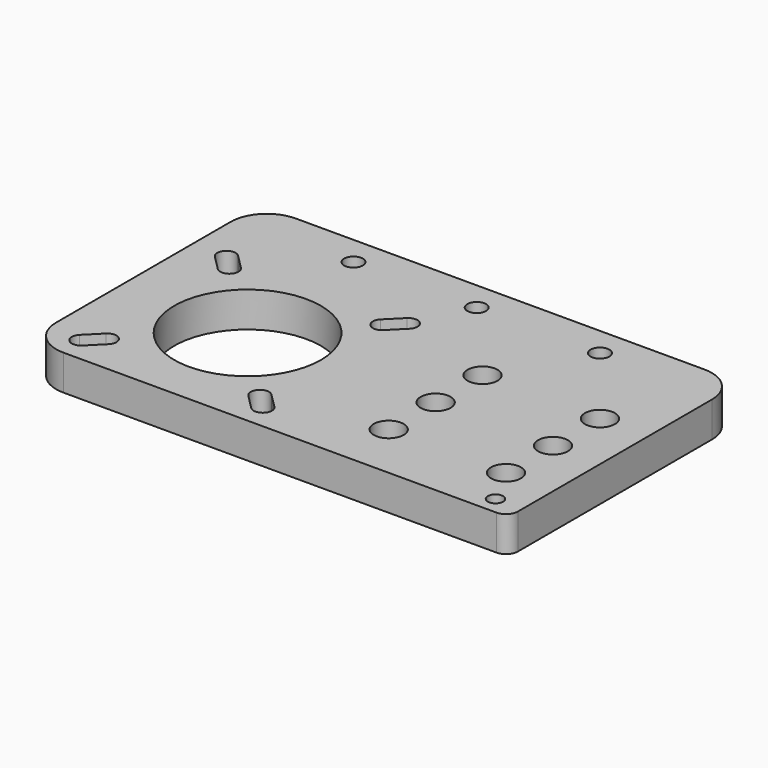
from build123d import *

# Parameters (mm, degrees)
F0_R     = 12.5
F0_R_2   = 2.55
F0_R_3   = 1.3
F0_R_4   = 1.6
F1_DEPTH = 6


# Not quite as in the source:
# - ends of sketch curves that miss each other by under 0.0002 mm in the source are joined


with BuildPart() as f1:
    # F0 (on Top) → F1 (new body)
    with BuildSketch(Plane.XY):
        with BuildLine():
            Line((34.83, 24.75), (-34.83, 24.75))
            ThreePointArc((-34.83, 24.75), (-39.1928488399, 22.9428488399), (-41, 18.58))
            Line((-41, 18.58), (-41, -18.58))
            ThreePointArc((-41, -18.58), (-39.1928488399, -22.9428488399), (-34.83, -24.75))
            Line((-34.83, -24.75), (39, -24.75))
            ThreePointArc((39, -24.75), (40.4142135624, -24.1642135624), (41, -22.75))
            Line((41, -22.75), (41, 18.58))
            ThreePointArc((41, 18.58), (39.1928488399, 22.9428488399), (34.83, 24.75))
        make_face()
        with BuildLine():
            ThreePointArc((-34.1539839892, -21.5960150108), (-36.3460155108, -21.5960155108), (-36.3460150108, -19.4039839892))
            Line((-36.346015, -19.403984), (-33.846015, -16.903984))
            ThreePointArc((-33.8460150108, -16.9039839892), (-31.6539844892, -16.9039844892), (-31.6539839892, -19.0960150108))
            Line((-31.653984, -19.096015), (-34.153984, -21.596015))
        make_face(mode=Mode.SUBTRACT)
        with BuildLine():
            ThreePointArc((-3.1539844892, -19.4039844892), (-3.1539844892, -21.5960155108), (-5.3460155108, -21.5960155108))
            Line((-5.3460155108, -21.5960155108), (-7.846015, -19.096015))
            ThreePointArc((-7.846015, -19.096015), (-7.8460155108, -16.9039844892), (-5.6539844892, -16.9039844892))
            Line((-5.6539844892, -16.9039844892), (-3.1539844892, -19.4039844892))
        make_face(mode=Mode.SUBTRACT)
        with Locations((-19.25, -5)):
            Circle(F0_R, mode=Mode.SUBTRACT)
        with Locations((12.8, -15)):
            Circle(F0_R_2, mode=Mode.SUBTRACT)
        with Locations((36.4, -21.75)):
            Circle(F0_R_3, mode=Mode.SUBTRACT)
        with Locations((32.8, -15)):
            Circle(F0_R_2, mode=Mode.SUBTRACT)
        with Locations((12.8, -5)):
            Circle(F0_R_2, mode=Mode.SUBTRACT)
        with Locations((32.8, -5)):
            Circle(F0_R_2, mode=Mode.SUBTRACT)
        with BuildLine():
            ThreePointArc((-31.6539844892, 9.0960155108), (-31.6539844892, 6.9039844892), (-33.8460155108, 6.9039844892))
            Line((-33.8460155108, 6.9039844892), (-36.346015, 9.403985))
            ThreePointArc((-36.346015, 9.403985), (-36.3460155108, 11.5960155108), (-34.1539844892, 11.5960155108))
            Line((-34.1539844892, 11.5960155108), (-31.6539844892, 9.0960155108))
        make_face(mode=Mode.SUBTRACT)
        with BuildLine():
            ThreePointArc((-5.3460150108, 11.5960160108), (-3.1539844892, 11.5960155108), (-3.1539839892, 9.4039849892))
            Line((-3.153984, 9.403985), (-5.653984, 6.903985))
            ThreePointArc((-5.6539839892, 6.9039849892), (-7.8460155108, 6.9039844892), (-7.8460150108, 9.0960160108))
            Line((-7.846015, 9.096016), (-5.346015, 11.596016))
        make_face(mode=Mode.SUBTRACT)
        with Locations((-21, 19.75)):
            Circle(F0_R_4, mode=Mode.SUBTRACT)
        with Locations((12.8, 5)):
            Circle(F0_R_2, mode=Mode.SUBTRACT)
        with Locations((32.8, 5)):
            Circle(F0_R_2, mode=Mode.SUBTRACT)
        with Locations((0, 19.75)):
            Circle(F0_R_4, mode=Mode.SUBTRACT)
        with Locations((21, 19.75)):
            Circle(F0_R_4, mode=Mode.SUBTRACT)
    extrude(amount=F1_DEPTH)


solid = f1.part
